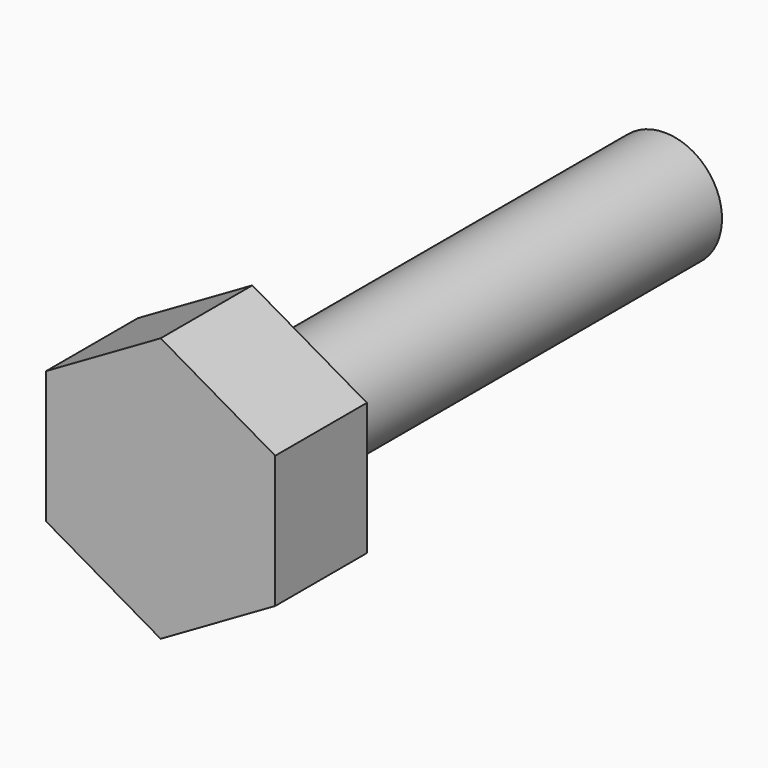
from build123d import *

# Parameters (mm, degrees)
F0_R     = 1
F1_DEPTH = 2
F2_R     = 1
F3_DEPTH = 9


# Not quite as in the source:
# - a feature of the source that left no trace in its solid (it failed there, or was rolled back) is left out


with BuildPart() as f1:
    # F0 (on Front) → F1 (new body)
    with BuildSketch(Plane.XZ):
        Polygon((-2, 1.1547005384), (-2, -1.1547005384), (0, -2.3094010768), (2, -1.1547005384), (2, 1.1547005384), (0, 2.3094010768), align=None)
        Circle(F0_R, mode=Mode.SUBTRACT)
        Circle(F0_R)
    extrude(amount=F1_DEPTH)

    # F2 (on face) → F3 (join)
    with BuildSketch(Plane(origin=(0, 0, 0), x_dir=(-1, 0, 0), z_dir=(0, 1, 0))):
        Circle(F2_R)
    extrude(amount=F3_DEPTH)


solid = f1.part
